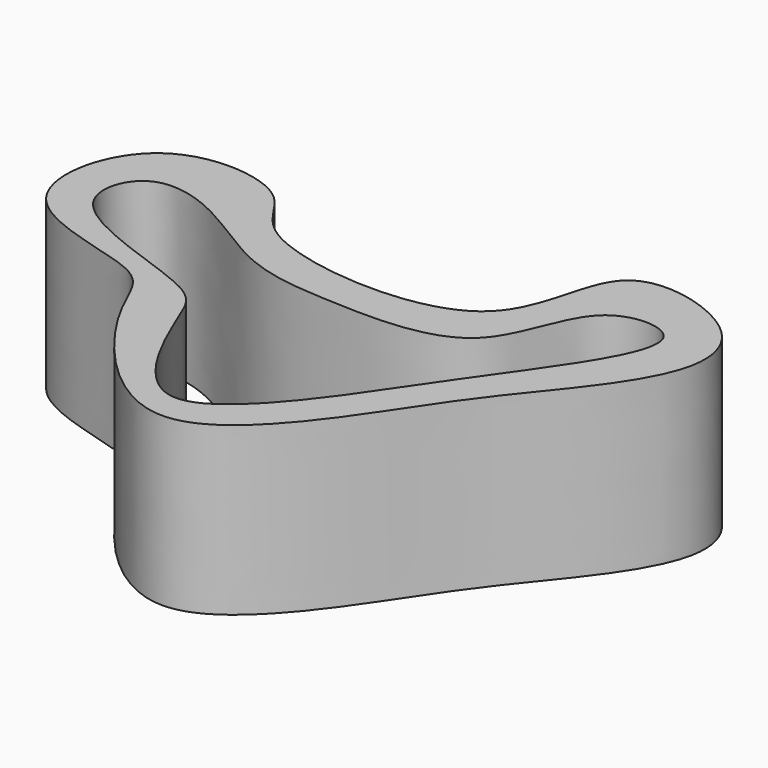
from build123d import *

# Parameters (mm, degrees)
F1_DEPTH = 25.4


with BuildPart() as f1:
    # F0 (on Top) → F1 (new body)
    with BuildSketch(Plane.XY):
        with BuildLine():
            add(Edge.make_bspline(
                [(-16.3379199803, 32.8285321593), (-20.3492653021, 35.2964883012), (-20.9996050024, 42.7931028363), (-43.7302335193, 45.0437331975), (-49.5672538017, 18.4634019032), (-21.7689804117, 16.4462415083), (-20.5577343748, 5.969968658), (3.498849019, -24.5194770021), (25.2687772703, 11.5287727158), (33.6686118545, 21.3937620323), (45.1099114539, 36.2598880766), (41.5311524262, 48.822454206), (18.4479088942, 54.8129506074), (21.8189275863, 25.6377721477), (-9.4939579424, 28.6178255781), (-16.3379199803, 32.8285321593)],
                knots=[0, 0, 0, 0, 0.0591328182, 0.1328628988, 0.208604586, 0.2911455319, 0.3489722945, 0.4436909786, 0.5447015421, 0.6159721837, 0.689500429, 0.7491920515, 0.8212976628, 0.8991104654, 1, 1, 1, 1], degree=3))
        make_face()
        with BuildLine():
            add(Edge.make_bspline(
                [(-14.5056303591, 25.804752484), (-10.1638023825, 23.9464410429), (-0.6082752719, 23.2057694489), (22.0897433333, 22.8343139859), (23.4966478871, 43.5204731705), (40.9479870997, 42.8049406687), (28.4928951554, 23.9863930061), (21.7938670664, 15.1228707357), (-0.3452540195, -18.8906637654), (-12.7322752056, 9.1320760206), (-14.9195105069, 16.2701054453), (-42.5493777905, 22.1511125152), (-38.4580661407, 36.1577589428), (-26.6021795012, 33.8723101193), (-18.8956538123, 27.6836916897), (-14.5056303591, 25.804752484)],
                knots=[0, 0, 0, 0, 0.0755572573, 0.1617333866, 0.24124179, 0.2998853883, 0.3783898248, 0.4572188479, 0.5633878245, 0.6508254669, 0.7090466222, 0.8050837026, 0.8619600393, 0.9236040365, 1, 1, 1, 1], degree=3))
        make_face(mode=Mode.SUBTRACT)
    extrude(amount=F1_DEPTH)


solid = f1.part
